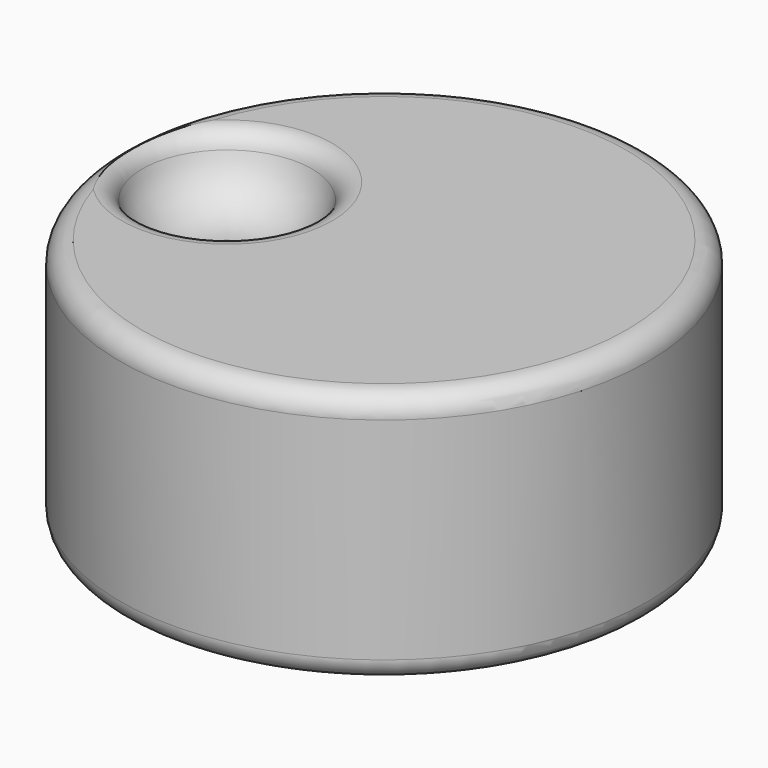
from build123d import *

# Parameters (mm, degrees)
F0_R     = 12.5
F0_R_2   = 3
F1_DEPTH = 10
F2_R     = 12.5
F2_R_2   = 3
F3_DEPTH = 2
F4_R     = 4.1082069006
F5_DEPTH = 3
F6_R     = 2.99999
F8_R     = 1
F9_SIZE  = 1


# Not quite as in the source:
# - a fillet or chamfer that OpenCascade refuses, or shapes differently, is made with other operations: its cross-section is extruded or revolved along the edge and cut away or added
# - a fillet or chamfer is up to 0.001 mm smaller than in the source, because OpenCascade refuses the exact size


with BuildPart() as f1:
    # F0 (on Top) → F1 (new body)
    with BuildSketch(Plane.XY):
        Circle(F0_R)
        Circle(F0_R_2, mode=Mode.SUBTRACT)
    extrude(amount=F1_DEPTH)

    # F2 (on face) → F3 (join)
    with BuildSketch(Plane.XY.offset(10)):
        Circle(F2_R)
        Circle(F2_R_2, mode=Mode.SUBTRACT)
        Circle(F2_R_2)
    extrude(amount=F3_DEPTH)

    # F4 (on face) → F5 (cut)
    with BuildSketch(Plane.XY.offset(12)):
        with Locations((-7.4370889924, 0)):
            Circle(F4_R)
    extrude(amount=-F5_DEPTH, mode=Mode.SUBTRACT)

    # F6 (radius 3 in the source; OpenCascade refuses exactly that, so slightly less here)
    f6_edges = [f1.edges().sort_by_distance(p)[0] for p in [
        (-11.545296, 0, 9),
    ]]
    fillet(f6_edges, radius=F6_R)

    # F7: fillet of radius 1 on 2 edges, made by hand

    # F7_s1 → F7_t2 (revolve, cut)
    with BuildSketch(Plane.XZ):
        with BuildLine():
            ThreePointArc((11.5, 12), (12.2071067812, 11.7071067812), (12.5, 11))
            Line((12.5, 11), (12.5, 12))
            Line((12.5, 12), (11.5, 12))
        make_face()
    revolve(axis=Axis((0, 0, 12), (0, 0, 1)), mode=Mode.SUBTRACT)

    # F7_s3 → F7_t4 (revolve, cut)
    with BuildSketch(Plane.XZ):
        with BuildLine():
            ThreePointArc((-3.4241428123, 11.249998125), (-3.0682696928, 11.7905688221), (-2.4558964916, 12))
            Line((-2.4558964916, 12), (-2.4558964916, 12.1))
            Line((-2.4558964916, 12.1), (-3.3288820918, 12.1))
            Line((-3.3288820918, 12.1), (-3.4288820918, 12))
            ThreePointArc((-3.4288820918, 12), (-3.4288820918, 11.99999), (-3.5209674443, 11.2749979375))
            Line((-3.5209674443, 11.2749979375), (-3.4241428123, 11.249998125))
        make_face()
    revolve(axis=Axis((-7.4370889924, 0, 12), (0, 0, 1)), mode=Mode.SUBTRACT)

    # F8
    f8_edges = [f1.edges().sort_by_distance(p)[0] for p in [
        (-12.5, 0, 0),
    ]]
    fillet(f8_edges, radius=F8_R)

    # F9
    f9_edges = [f1.edges().sort_by_distance(p)[0] for p in [
        (-3, 0, 0),
    ]]
    chamfer(f9_edges, length=F9_SIZE)


solid = f1.part
